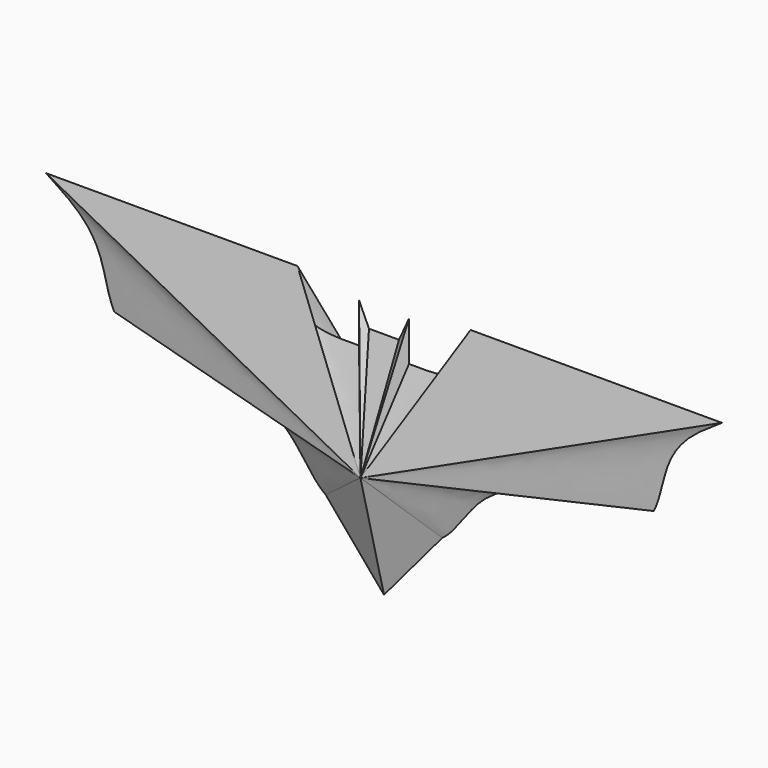
from build123d import *


with BuildPart() as f3:
    # F0 (on Front) → F3 section 0
    with BuildSketch(Plane.XZ, mode=Mode.PRIVATE) as f3_s0:
        with BuildLine():
            Line((-21.9142735004, 32.6593369246), (-64.6117627621, 32.6593369246))
            add(Edge.make_bspline(
                [(-64.6117627621, 32.6593369246), (-63.1112154786, 31.6044133494), (-59.4897111338, 29.4798106269), (-54.8402694545, 24.0083886157), (-54.1776311477, 17.803548493), (-53.0184023082, 15.6934484839)],
                knots=[0, 0, 0, 0, 0.3044179075, 0.6380886555, 1, 1, 1, 1], degree=3))
            add(Edge.make_bspline(
                [(-53.0184023082, 15.6934484839), (-50.397152359, 15.9517944961), (-42.4564652069, 16.5735141568), (-30.3318480055, 11.9726995365), (-22.6326325716, 7.7807102957), (-19.3285813991, 1.5879180834), (-17.1072725207, 0)],
                knots=[0, 0, 0, 0, 0.2494885994, 0.5320392712, 0.7637954486, 1, 1, 1, 1], degree=3))
            Line((-17.1072725207, 0), (-7.2105028667, -11.7347398773))
            Line((-7.2105028667, -11.7347398773), (2.6862667874, 0))
            add(Edge.make_bspline(
                [(38.5973965749, 15.6934484839), (35.9761466257, 15.9517944961), (28.0354594736, 16.5735141568), (15.9108422722, 11.9726995365), (8.2116268383, 7.7807102957), (4.9075756658, 1.5879180834), (2.6862667874, 0)],
                knots=[0, 0, 0, 0, 0.2494885994, 0.5320392712, 0.7637954486, 1, 1, 1, 1], degree=3))
            add(Edge.make_bspline(
                [(50.1907570288, 32.6593369246), (48.6902097453, 31.6044133494), (45.0687054005, 29.4798106269), (40.4192637212, 24.0083886157), (39.7566254144, 17.803548493), (38.5973965749, 15.6934484839)],
                knots=[0, 0, 0, 0, 0.3044179075, 0.6380886555, 1, 1, 1, 1], degree=3))
            Line((50.1907570288, 32.6593369246), (7.4932677671, 32.6593369246))
            add(Edge.make_bspline(
                [(7.4932677671, 32.6593369246), (7.7789275206, 30.681626577), (8.3182882425, 26.9541985329), (4.3276740221, 24.1005648406), (-0.3013873529, 24.1408897918), (-2.9690302908, 24.1763927042)],
                knots=[0, 0, 0, 0, 0.3305961482, 0.6143190537, 1, 1, 1, 1], degree=3))
            Line((-2.9690302908, 24.1763927042), (-2.9690302908, 30.962748453))
            Line((-2.9690302908, 30.962748453), (-4.662130028, 27.2415857762))
            Line((-4.662130028, 27.2415857762), (-7.2105028667, 27.2415857762))
            Line((-7.2105028667, 27.2415857762), (-9.7588757053, 27.2415857762))
            Line((-9.7588757053, 27.2415857762), (-11.4519754425, 30.962748453))
            Line((-11.4519754425, 30.962748453), (-11.4519754425, 24.1763927042))
            add(Edge.make_bspline(
                [(-21.9142735004, 32.6593369246), (-22.199933254, 30.681626577), (-22.7392939758, 26.9541985329), (-18.7486797554, 24.1005648406), (-14.1196183804, 24.1408897918), (-11.4519754425, 24.1763927042)],
                knots=[0, 0, 0, 0, 0.3305961482, 0.6143190537, 1, 1, 1, 1], degree=3))
        make_face()
    loft([f3_s0.sketch, Vertex(-7.2105028667, -5, 7.7760326676)])

    # F0 (on Front) → F6 section 0
    with BuildSketch(Plane.XZ, mode=Mode.PRIVATE) as f6_s0:
        with BuildLine():
            Line((-21.9142735004, 32.6593369246), (-64.6117627621, 32.6593369246))
            add(Edge.make_bspline(
                [(-64.6117627621, 32.6593369246), (-63.1112154786, 31.6044133494), (-59.4897111338, 29.4798106269), (-54.8402694545, 24.0083886157), (-54.1776311477, 17.803548493), (-53.0184023082, 15.6934484839)],
                knots=[0, 0, 0, 0, 0.3044179075, 0.6380886555, 1, 1, 1, 1], degree=3))
            add(Edge.make_bspline(
                [(-53.0184023082, 15.6934484839), (-50.397152359, 15.9517944961), (-42.4564652069, 16.5735141568), (-30.3318480055, 11.9726995365), (-22.6326325716, 7.7807102957), (-19.3285813991, 1.5879180834), (-17.1072725207, 0)],
                knots=[0, 0, 0, 0, 0.2494885994, 0.5320392712, 0.7637954486, 1, 1, 1, 1], degree=3))
            Line((-17.1072725207, 0), (-7.2105028667, -11.7347398773))
            Line((-7.2105028667, -11.7347398773), (2.6862667874, 0))
            add(Edge.make_bspline(
                [(38.5973965749, 15.6934484839), (35.9761466257, 15.9517944961), (28.0354594736, 16.5735141568), (15.9108422722, 11.9726995365), (8.2116268383, 7.7807102957), (4.9075756658, 1.5879180834), (2.6862667874, 0)],
                knots=[0, 0, 0, 0, 0.2494885994, 0.5320392712, 0.7637954486, 1, 1, 1, 1], degree=3))
            add(Edge.make_bspline(
                [(50.1907570288, 32.6593369246), (48.6902097453, 31.6044133494), (45.0687054005, 29.4798106269), (40.4192637212, 24.0083886157), (39.7566254144, 17.803548493), (38.5973965749, 15.6934484839)],
                knots=[0, 0, 0, 0, 0.3044179075, 0.6380886555, 1, 1, 1, 1], degree=3))
            Line((50.1907570288, 32.6593369246), (7.4932677671, 32.6593369246))
            add(Edge.make_bspline(
                [(7.4932677671, 32.6593369246), (7.7789275206, 30.681626577), (8.3182882425, 26.9541985329), (4.3276740221, 24.1005648406), (-0.3013873529, 24.1408897918), (-2.9690302908, 24.1763927042)],
                knots=[0, 0, 0, 0, 0.3305961482, 0.6143190537, 1, 1, 1, 1], degree=3))
            Line((-2.9690302908, 24.1763927042), (-2.9690302908, 30.962748453))
            Line((-2.9690302908, 30.962748453), (-4.662130028, 27.2415857762))
            Line((-4.662130028, 27.2415857762), (-7.2105028667, 27.2415857762))
            Line((-7.2105028667, 27.2415857762), (-9.7588757053, 27.2415857762))
            Line((-9.7588757053, 27.2415857762), (-11.4519754425, 30.962748453))
            Line((-11.4519754425, 30.962748453), (-11.4519754425, 24.1763927042))
            add(Edge.make_bspline(
                [(-21.9142735004, 32.6593369246), (-22.199933254, 30.681626577), (-22.7392939758, 26.9541985329), (-18.7486797554, 24.1005648406), (-14.1196183804, 24.1408897918), (-11.4519754425, 24.1763927042)],
                knots=[0, 0, 0, 0, 0.3305961482, 0.6143190537, 1, 1, 1, 1], degree=3))
        make_face()
    loft([f6_s0.sketch, Vertex(-7.2105028667, 5, 7.7760326676)])


solid = f3.part
